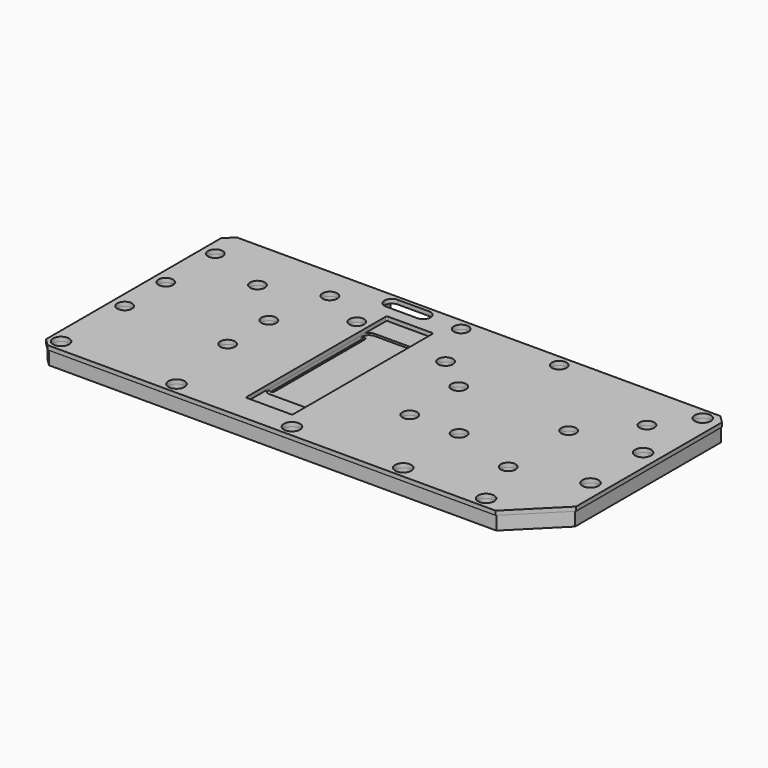
from build123d import *

# Parameters (mm, degrees)
F0_R     = 1.75
F0_R_2   = 1.6
F0_W     = 33.35
F0_H     = 3.8
F1_DEPTH = 0.9
F2_R     = 1.75
F2_R_2   = 1.6
F3_DEPTH = 3
F4_DEPTH = 0.45
F5_DEPTH = 0.9


# Not quite as in the source:
# - after a boolean that leaves OpenCascade's solid faulty, fix() repairs it
# - ends of sketch curves that miss each other by under 0.0002 mm in the source are joined


with BuildPart() as f1:
    # F0 (on Top) → F1 (new body)
    with BuildSketch(Plane.XY):
        Polygon((-54.3477, 23.6), (-54.3477, -23.95), (-52.7977, -25.5), (44.6523, -25.5), (54.3523, -15.8), (54.3523, 23.85), (52.7023, 25.5), (-52.4477, 25.5), align=None)
        with Locations((-51.8477, -23)):
            Circle(F0_R, mode=Mode.SUBTRACT)
        with Locations((-26.7477, -23)):
            Circle(F0_R, mode=Mode.SUBTRACT)
        with Locations((-1.6477, -23)):
            Circle(F0_R, mode=Mode.SUBTRACT)
        with Locations((-51.5477, -6.1)):
            Circle(F0_R_2, mode=Mode.SUBTRACT)
        with Locations((-29.1477, -6.1)):
            Circle(F0_R_2, mode=Mode.SUBTRACT)
        with BuildLine():
            Line((-14.4977, -19.28), (-14.4977, 18.54))
            ThreePointArc((-14.4977, 18.54), (-14.4215477631, 18.7238477631), (-14.2377, 18.8))
            Line((-14.2377, 18.8), (-4.5977, 18.8))
            ThreePointArc((-4.5977, 18.8), (-4.4138515904, 18.7238481167), (-4.337699, 18.54))
            Line((-4.337699, 18.54), (-4.3377, -19.28))
            ThreePointArc((-4.3377, -19.28), (-4.4138515904, -19.4638481167), (-4.5977, -19.54))
            Line((-4.5977, -19.54), (-14.2377, -19.54))
            ThreePointArc((-14.2377, -19.54), (-14.4215477631, -19.4638477631), (-14.4977, -19.28))
        make_face(mode=Mode.SUBTRACT)
        with Locations((22.5523, -23)):
            Circle(F0_R, mode=Mode.SUBTRACT)
        with Locations((40.5523, -23)):
            Circle(F0_R, mode=Mode.SUBTRACT)
        with Locations((11.2523, -7.1)):
            Circle(F0_R_2, mode=Mode.SUBTRACT)
        with Locations((22.0523, -7.2)):
            Circle(F0_R_2, mode=Mode.SUBTRACT)
        with Locations((36.2523, -11.6)):
            Circle(F0_R_2, mode=Mode.SUBTRACT)
        with Locations((50.8523, -7.5)):
            Circle(F0_R, mode=Mode.SUBTRACT)
        with Locations((-51.5477, 5.1)):
            Circle(F0_R_2, mode=Mode.SUBTRACT)
        with Locations((-29.1477, 5.1)):
            Circle(F0_R_2, mode=Mode.SUBTRACT)
        with Locations((-51.5477, 18.55)):
            Circle(F0_R_2, mode=Mode.SUBTRACT)
        with Locations((-38.7477, 14)):
            Circle(F0_R_2, mode=Mode.SUBTRACT)
        with Locations((-36.035871, 22.938344)):
            Rectangle(F0_W, F0_H, mode=Mode.SUBTRACT)
        with Locations((-17.1477, 14)):
            Circle(F0_R_2, mode=Mode.SUBTRACT)
        with Locations((-26.6477, 18.55)):
            Circle(F0_R_2, mode=Mode.SUBTRACT)
        with BuildLine():
            ThreePointArc((-16.7667, 21.4529), (-17.8980708499, 21.9215291501), (-18.3667, 23.0529))
            ThreePointArc((-18.3667, 23.0529), (-17.8980708499, 24.1842708499), (-16.7667, 24.6529))
            Line((-16.7667, 24.6529), (-9.9667, 24.6529))
            ThreePointArc((-9.9667, 24.6529), (-8.8353291501, 24.1842708499), (-8.3667, 23.0529))
            ThreePointArc((-8.3667, 23.0529), (-8.8353291501, 21.9215291501), (-9.9667, 21.4529))
            Line((-9.9667, 21.4529), (-16.7667, 21.4529))
        make_face(mode=Mode.SUBTRACT)
        with Locations((-1.6477, 23)):
            Circle(F0_R_2, mode=Mode.SUBTRACT)
        with Locations((11.2523, 6.2)):
            Circle(F0_R_2, mode=Mode.SUBTRACT)
        with Locations((3.7523, 12)):
            Circle(F0_R_2, mode=Mode.SUBTRACT)
        with Locations((35.9523, 5.2)):
            Circle(F0_R_2, mode=Mode.SUBTRACT)
        with Locations((50.8523, 6.8)):
            Circle(F0_R, mode=Mode.SUBTRACT)
        with Locations((19.6523, 23)):
            Circle(F0_R_2, mode=Mode.SUBTRACT)
        with Locations((45.0523, 15.1)):
            Circle(F0_R_2, mode=Mode.SUBTRACT)
        with Locations((50.8523, 23)):
            Circle(F0_R, mode=Mode.SUBTRACT)
        with Locations((-36.035871, 22.938344)):
            Rectangle(F0_W, F0_H)
    extrude(amount=F1_DEPTH)


with BuildPart() as f3:
    # F2 (on Top) → F3 (new body)
    with BuildSketch(Plane.XY):
        with BuildLine():
            ThreePointArc((-17.36885, 21.2528), (-18.4295101718, 21.6921398282), (-18.86885, 22.7528))
            Line((-18.86885, 22.7528), (-18.86885, 25.2999))
            Line((-18.86885, 25.2999), (-52.25015, 25.2999))
            Line((-52.25015, 25.2999), (-54.15015, 23.3999))
            Line((-54.15015, 23.3999), (-54.15015, -23.7999))
            Line((-54.15015, -23.7999), (-52.65015, -25.2999))
            Line((-52.65015, -25.2999), (44.65015, -25.2999))
            Line((44.65015, -25.2999), (54.15015, -15.7999))
            Line((54.15015, -15.7999), (54.15015, 23.7999))
            Line((54.15015, 23.7999), (52.65015, 25.2999))
            Line((52.65015, 25.2999), (-7.86885, 25.2999))
            Line((-7.86885, 25.2999), (-7.86885, 22.7528))
            ThreePointArc((-7.86885, 22.7528), (-8.3081898282, 21.6921398282), (-9.36885, 21.2528))
            Line((-9.36885, 21.2528), (-17.36885, 21.2528))
        make_face()
        with Locations((-51.84985, -23.0001)):
            Circle(F2_R, mode=Mode.SUBTRACT)
        with Locations((-26.74985, -23.0001)):
            Circle(F2_R, mode=Mode.SUBTRACT)
        with Locations((-1.64985, -23.0001)):
            Circle(F2_R, mode=Mode.SUBTRACT)
        with Locations((-51.54985, -6.1001)):
            Circle(F2_R_2, mode=Mode.SUBTRACT)
        with Locations((-29.14985, -6.1001)):
            Circle(F2_R_2, mode=Mode.SUBTRACT)
        with BuildLine():
            Line((-14.62685, 11.8049), (-14.62685, 12.3049))
            ThreePointArc((-14.62685, 12.3049), (-14.1875101718, 13.3655601718), (-13.12685, 13.8049))
            Line((-13.12685, 13.8049), (-5.72685, 13.8049))
            ThreePointArc((-5.72685, 13.8049), (-4.6661898282, 13.3655601718), (-4.22685, 12.3049))
            Line((-4.22685, 12.3049), (-4.22685, 11.8049))
            Line((-4.22685, 11.8049), (-4.22685, -12.6951))
            Line((-4.22685, -12.6951), (-4.22685, -13.1951))
            ThreePointArc((-4.22685, -13.1951), (-4.6661898282, -14.2557601718), (-5.72685, -14.6951))
            Line((-5.72685, -14.6951), (-13.12685, -14.6951))
            ThreePointArc((-13.12685, -14.6951), (-14.1875101718, -14.2557601718), (-14.62685, -13.1951))
            Line((-14.62685, -13.1951), (-14.62685, -12.6951))
            Line((-14.62685, -12.6951), (-14.62685, 11.8049))
        make_face(mode=Mode.SUBTRACT)
        with Locations((22.55015, -23.0001)):
            Circle(F2_R, mode=Mode.SUBTRACT)
        with Locations((40.55015, -23.0001)):
            Circle(F2_R, mode=Mode.SUBTRACT)
        with Locations((11.25015, -7.1001)):
            Circle(F2_R_2, mode=Mode.SUBTRACT)
        with Locations((22.05015, -7.2001)):
            Circle(F2_R_2, mode=Mode.SUBTRACT)
        with Locations((36.25015, -11.6001)):
            Circle(F2_R_2, mode=Mode.SUBTRACT)
        with Locations((50.85015, -7.5001)):
            Circle(F2_R, mode=Mode.SUBTRACT)
        with Locations((-51.54985, 5.0999)):
            Circle(F2_R_2, mode=Mode.SUBTRACT)
        with Locations((-29.14985, 5.0999)):
            Circle(F2_R_2, mode=Mode.SUBTRACT)
        with Locations((-51.54985, 18.5499)):
            Circle(F2_R_2, mode=Mode.SUBTRACT)
        with Locations((-38.74985, 13.9999)):
            Circle(F2_R_2, mode=Mode.SUBTRACT)
        with Locations((-17.14985, 13.9999)):
            Circle(F2_R_2, mode=Mode.SUBTRACT)
        with Locations((-26.64985, 18.5499)):
            Circle(F2_R_2, mode=Mode.SUBTRACT)
        with Locations((-1.64985, 22.9999)):
            Circle(F2_R_2, mode=Mode.SUBTRACT)
        with Locations((11.25015, 6.1999)):
            Circle(F2_R_2, mode=Mode.SUBTRACT)
        with Locations((3.75015, 11.9999)):
            Circle(F2_R_2, mode=Mode.SUBTRACT)
        with Locations((35.95015, 5.1999)):
            Circle(F2_R_2, mode=Mode.SUBTRACT)
        with Locations((50.85015, 6.7999)):
            Circle(F2_R, mode=Mode.SUBTRACT)
        with Locations((19.65015, 22.9999)):
            Circle(F2_R_2, mode=Mode.SUBTRACT)
        with Locations((45.05015, 15.0999)):
            Circle(F2_R_2, mode=Mode.SUBTRACT)
        with Locations((50.85015, 22.9999)):
            Circle(F2_R, mode=Mode.SUBTRACT)
        with BuildLine():
            ThreePointArc((-13.12685, 13.8049), (-14.1875101718, 13.3655601718), (-14.62685, 12.3049))
            Line((-14.62685, 12.3049), (-14.62685, 11.8049))
            ThreePointArc((-14.62685, 11.8049), (-14.4804033906, 12.1584533906), (-14.12685, 12.3049))
            ThreePointArc((-14.12685, 12.3049), (-13.7732966094, 12.1584533906), (-13.62685, 11.8049))
            Line((-13.62685, 11.8049), (-13.62685, -12.6951))
            ThreePointArc((-13.62685, -12.6951), (-13.7732966094, -13.0486533906), (-14.12685, -13.1951))
            ThreePointArc((-14.12685, -13.1951), (-14.4804033906, -13.0486533906), (-14.62685, -12.6951))
            Line((-14.62685, -12.6951), (-14.62685, -13.1951))
            ThreePointArc((-14.62685, -13.1951), (-14.1875101718, -14.2557601718), (-13.12685, -14.6951))
            Line((-13.12685, -14.6951), (-5.72685, -14.6951))
            ThreePointArc((-5.72685, -14.6951), (-4.6661898282, -14.2557601718), (-4.22685, -13.1951))
            Line((-4.22685, -13.1951), (-4.22685, -12.6951))
            ThreePointArc((-4.22685, -12.6951), (-4.3732966094, -13.0486533906), (-4.72685, -13.1951))
            ThreePointArc((-4.72685, -13.1951), (-5.0804033906, -13.0486533906), (-5.22685, -12.6951))
            Line((-5.22685, -12.6951), (-5.22685, 11.8049))
            ThreePointArc((-5.22685, 11.8049), (-5.0804033906, 12.1584533906), (-4.72685, 12.3049))
            ThreePointArc((-4.72685, 12.3049), (-4.3732966094, 12.1584533906), (-4.22685, 11.8049))
            Line((-4.22685, 11.8049), (-4.22685, 12.3049))
            ThreePointArc((-4.22685, 12.3049), (-4.6661898282, 13.3655601718), (-5.72685, 13.8049))
            Line((-5.72685, 13.8049), (-13.12685, 13.8049))
        make_face()
        with BuildLine():
            ThreePointArc((-14.12685, 12.3049), (-14.4804033906, 12.1584533906), (-14.62685, 11.8049))
            Line((-14.62685, 11.8049), (-14.62685, -12.6951))
            ThreePointArc((-14.62685, -12.6951), (-14.4804033906, -13.0486533906), (-14.12685, -13.1951))
            ThreePointArc((-14.12685, -13.1951), (-13.7732966094, -13.0486533906), (-13.62685, -12.6951))
            Line((-13.62685, -12.6951), (-13.62685, 11.8049))
            ThreePointArc((-13.62685, 11.8049), (-13.7732966094, 12.1584533906), (-14.12685, 12.3049))
        make_face()
        with BuildLine():
            Line((-4.22685, -12.6951), (-4.22685, 11.8049))
            ThreePointArc((-4.22685, 11.8049), (-4.3732966094, 12.1584533906), (-4.72685, 12.3049))
            ThreePointArc((-4.72685, 12.3049), (-5.0804033906, 12.1584533906), (-5.22685, 11.8049))
            Line((-5.22685, 11.8049), (-5.22685, -12.6951))
            ThreePointArc((-5.22685, -12.6951), (-5.0804033906, -13.0486533906), (-4.72685, -13.1951))
            ThreePointArc((-4.72685, -13.1951), (-4.3732966094, -13.0486533906), (-4.22685, -12.6951))
        make_face()
    extrude(amount=-F3_DEPTH)

    # F2 (on Top) → F4 (cut)
    with BuildSketch(Plane.XY):
        with BuildLine():
            ThreePointArc((-13.12685, 13.8049), (-14.1875101718, 13.3655601718), (-14.62685, 12.3049))
            Line((-14.62685, 12.3049), (-14.62685, 11.8049))
            ThreePointArc((-14.62685, 11.8049), (-14.4804033906, 12.1584533906), (-14.12685, 12.3049))
            ThreePointArc((-14.12685, 12.3049), (-13.7732966094, 12.1584533906), (-13.62685, 11.8049))
            Line((-13.62685, 11.8049), (-13.62685, -12.6951))
            ThreePointArc((-13.62685, -12.6951), (-13.7732966094, -13.0486533906), (-14.12685, -13.1951))
            ThreePointArc((-14.12685, -13.1951), (-14.4804033906, -13.0486533906), (-14.62685, -12.6951))
            Line((-14.62685, -12.6951), (-14.62685, -13.1951))
            ThreePointArc((-14.62685, -13.1951), (-14.1875101718, -14.2557601718), (-13.12685, -14.6951))
            Line((-13.12685, -14.6951), (-5.72685, -14.6951))
            ThreePointArc((-5.72685, -14.6951), (-4.6661898282, -14.2557601718), (-4.22685, -13.1951))
            Line((-4.22685, -13.1951), (-4.22685, -12.6951))
            ThreePointArc((-4.22685, -12.6951), (-4.3732966094, -13.0486533906), (-4.72685, -13.1951))
            ThreePointArc((-4.72685, -13.1951), (-5.0804033906, -13.0486533906), (-5.22685, -12.6951))
            Line((-5.22685, -12.6951), (-5.22685, 11.8049))
            ThreePointArc((-5.22685, 11.8049), (-5.0804033906, 12.1584533906), (-4.72685, 12.3049))
            ThreePointArc((-4.72685, 12.3049), (-4.3732966094, 12.1584533906), (-4.22685, 11.8049))
            Line((-4.22685, 11.8049), (-4.22685, 12.3049))
            ThreePointArc((-4.22685, 12.3049), (-4.6661898282, 13.3655601718), (-5.72685, 13.8049))
            Line((-5.72685, 13.8049), (-13.12685, 13.8049))
        make_face()
    extrude(amount=-F4_DEPTH, mode=Mode.SUBTRACT)

    # F2 (on Top) → F5 (cut)
    with BuildSketch(Plane.XY):
        with BuildLine():
            ThreePointArc((-14.12685, 12.3049), (-14.4804033906, 12.1584533906), (-14.62685, 11.8049))
            Line((-14.62685, 11.8049), (-14.62685, -12.6951))
            ThreePointArc((-14.62685, -12.6951), (-14.4804033906, -13.0486533906), (-14.12685, -13.1951))
            ThreePointArc((-14.12685, -13.1951), (-13.7732966094, -13.0486533906), (-13.62685, -12.6951))
            Line((-13.62685, -12.6951), (-13.62685, 11.8049))
            ThreePointArc((-13.62685, 11.8049), (-13.7732966094, 12.1584533906), (-14.12685, 12.3049))
        make_face()
        with BuildLine():
            Line((-4.22685, -12.6951), (-4.22685, 11.8049))
            ThreePointArc((-4.22685, 11.8049), (-4.3732966094, 12.1584533906), (-4.72685, 12.3049))
            ThreePointArc((-4.72685, 12.3049), (-5.0804033906, 12.1584533906), (-5.22685, 11.8049))
            Line((-5.22685, 11.8049), (-5.22685, -12.6951))
            ThreePointArc((-5.22685, -12.6951), (-5.0804033906, -13.0486533906), (-4.72685, -13.1951))
            ThreePointArc((-4.72685, -13.1951), (-4.3732966094, -13.0486533906), (-4.22685, -12.6951))
        make_face()
    extrude(amount=-F5_DEPTH, mode=Mode.SUBTRACT)

    add(f3.part.fix(), mode=Mode.REPLACE)


solid = Compound([f1.part, f3.part])
